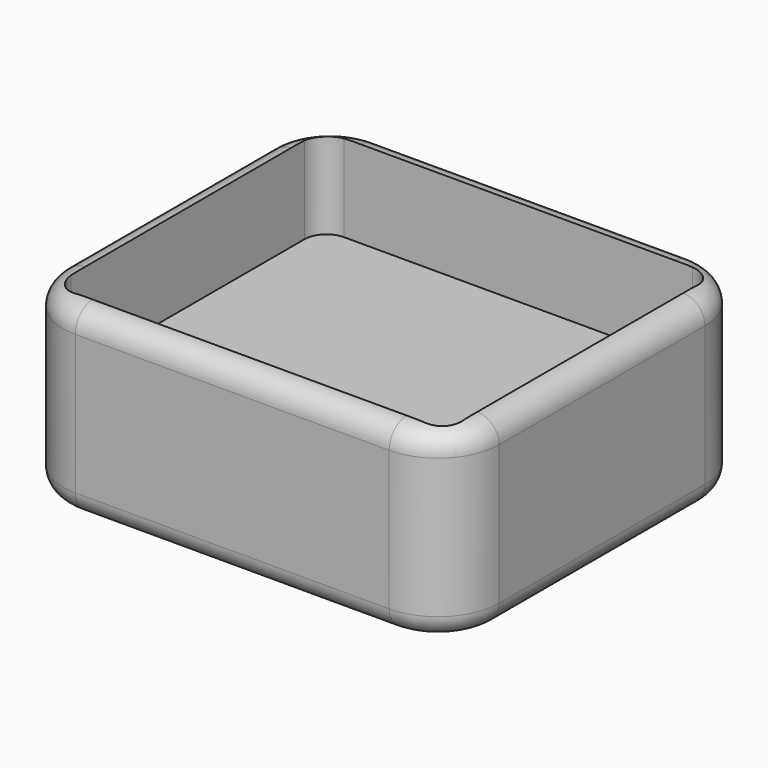
from build123d import *

# Parameters (mm, degrees)
F0_W         = 90
F0_H         = 77
F1_DEPTH     = 22
F0_W_2       = 100
F0_H_2       = 87
F2_DEPTH     = 42
F3_R         = 14
F4_R         = 5
F5_R         = 5
F6_T1_DEPTH  = 72
F6_T3_DEPTH  = 59
F6_T6_ANGLE  = 90
F6_T8_ANGLE  = 90
F6_T10_ANGLE = 90
F6_T12_ANGLE = 90


# Not quite as in the source:
# - a fillet or chamfer that OpenCascade refuses, or shapes differently, is made with other operations: its cross-section is extruded or revolved along the edge and cut away or added


with BuildPart() as f1:
    # F0 (on Top) → F1 (new body)
    with BuildSketch(Plane.XY):
        Rectangle(F0_W, F0_H)
    extrude(amount=F1_DEPTH)

    # F0 (on Top) → F2 (join)
    with BuildSketch(Plane.XY):
        Rectangle(F0_W_2, F0_H_2)
        Rectangle(F0_W, F0_H, mode=Mode.SUBTRACT)
    extrude(amount=F2_DEPTH)

    # F3
    f3_edges = [f1.edges().sort_by_distance(p)[0] for p in [
        (-50, -43.5, 21),
        (-50, 43.5, 21),
        (50, 43.5, 21),
        (50, -43.5, 21),
    ]]
    fillet(f3_edges, radius=F3_R)

    # F4
    f4_edges = [f1.edges().sort_by_distance(p)[0] for p in [
        (0, 43.5, 0),
    ]]
    fillet(f4_edges, radius=F4_R)

    # F5
    f5_edges = [f1.edges().sort_by_distance(p)[0] for p in [
        (-45, -38.5, 32),
        (45, -38.5, 32),
        (-45, 38.5, 32),
        (45, 38.5, 32),
    ]]
    fillet(f5_edges, radius=F5_R)

    # F6: fillet of radius 5 on 8 edges, made by hand

    # F6_s2 → F6_t1 (cut)
    with BuildSketch(Plane.YZ.offset(-36)):
        with BuildLine():
            ThreePointArc((-38.5, 42), (-42.0355339059, 40.5355339059), (-43.5, 37))
            Line((-43.5, 37), (-43.5, 42))
            Line((-43.5, 42), (-38.5, 42))
        make_face()
        with BuildLine():
            ThreePointArc((38.5, 42), (42.0355339059, 40.5355339059), (43.5, 37))
            Line((43.5, 37), (43.5, 42))
            Line((43.5, 42), (38.5, 42))
        make_face()
    extrude(amount=F6_T1_DEPTH, mode=Mode.SUBTRACT)

    # F6_s4 → F6_t3 (cut)
    with BuildSketch(Plane.XZ.offset(-29.5)):
        with BuildLine():
            ThreePointArc((45, 42), (48.5355339059, 40.5355339059), (50, 37))
            Line((50, 37), (50, 42))
            Line((50, 42), (45, 42))
        make_face()
        with BuildLine():
            ThreePointArc((-45, 42), (-48.5355339059, 40.5355339059), (-50, 37))
            Line((-50, 37), (-50, 42))
            Line((-50, 42), (-45, 42))
        make_face()
    extrude(amount=F6_T3_DEPTH, mode=Mode.SUBTRACT)

    # F6_s5 → F6_t6 (revolve, cut)
    with BuildSketch(Plane.XZ.offset(29.5)):
        with BuildLine():
            ThreePointArc((45, 42), (48.5355339059, 40.5355339059), (50, 37))
            Line((50, 37), (50, 42))
            Line((50, 42), (45, 42))
        make_face()
    revolve(axis=Axis((36, -29.5, 42), (0, 0, -1)), revolution_arc=F6_T6_ANGLE, mode=Mode.SUBTRACT)

    # F6_s7 → F6_t8 (revolve, cut)
    with BuildSketch(Plane.XZ.offset(-29.5)):
        with BuildLine():
            ThreePointArc((45, 42), (48.5355339059, 40.5355339059), (50, 37))
            Line((50, 37), (50, 42))
            Line((50, 42), (45, 42))
        make_face()
    revolve(axis=Axis((36, 29.5, 42), (0, 0, 1)), revolution_arc=F6_T8_ANGLE, mode=Mode.SUBTRACT)

    # F6_s9 → F6_t10 (revolve, cut)
    with BuildSketch(Plane.XZ.offset(29.5)):
        with BuildLine():
            ThreePointArc((-45, 42), (-48.5355339059, 40.5355339059), (-50, 37))
            Line((-50, 37), (-50, 42))
            Line((-50, 42), (-45, 42))
        make_face()
    revolve(axis=Axis((-36, -29.5, 42), (0, 0, 1)), revolution_arc=F6_T10_ANGLE, mode=Mode.SUBTRACT)

    # F6_s11 → F6_t12 (revolve, cut)
    with BuildSketch(Plane.YZ.offset(-36)):
        with BuildLine():
            ThreePointArc((38.5, 42), (42.0355339059, 40.5355339059), (43.5, 37))
            Line((43.5, 37), (43.5, 42))
            Line((43.5, 42), (38.5, 42))
        make_face()
    revolve(axis=Axis((-36, 29.5, 42), (0, 0, 1)), revolution_arc=F6_T12_ANGLE, mode=Mode.SUBTRACT)


solid = f1.part
